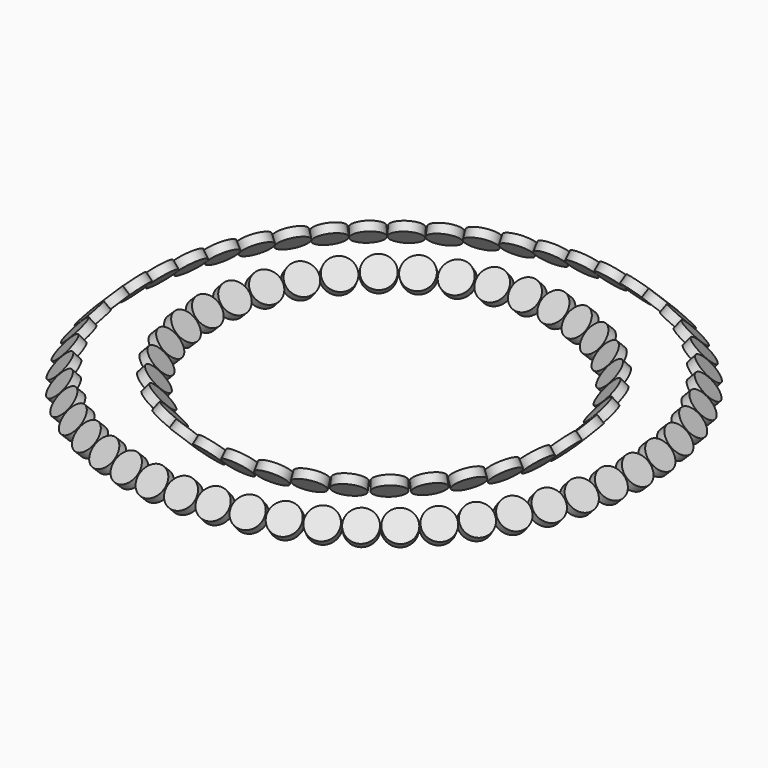
from build123d import *

# Parameters (mm, degrees)
F4_COUNT = 36
F5_COUNT = 52


# Not quite as in the source:
# - the program builds the solid bodies; features that only make, move or delete a surface that nothing else refers to are left out


with BuildPart() as f2:
    # F0 (on Front) → F2 (revolve)
    with BuildSketch(Plane.XZ):
        Polygon((-84.6237436867, 5.7022600949), (-88.1592775926, 2.166726189), (-86.9925514037, 1), (-83.4570174977, 4.5355339059), align=None)
        Polygon((-89.1138717472, 3.1213203436), (-88.1592775926, 2.166726189), (-84.6237436867, 5.7022600949), (-85.5783378413, 6.6568542495), align=None)
    revolve(axis=Axis((-84.0403805922, 0, 5.1188970004), (-0.7071067812, 0, 0.7071067812)))


with BuildPart() as f3:
    # F0 (on Front) → F3 (revolve)
    with BuildSketch(Plane.XZ):
        Polygon((-58.0074485963, 1), (-56.8407224074, 2.166726189), (-60.3762563133, 5.7022600949), (-61.5429825023, 4.5355339059), align=None)
        Polygon((-60.3762563133, 5.7022600949), (-56.8407224074, 2.166726189), (-55.8861282528, 3.1213203436), (-59.4216621587, 6.6568542495), align=None)
    revolve(axis=Axis((-60.9596194078, 0, 5.1188970004), (0.7071067812, 0, 0.7071067812)))


with BuildPart() as f4_1:
    # F4: instance of F3
    add(f3.part.rotate(Axis((0, 0, 16.5421869606), (0, 0, 1)), 1 * 360 / F4_COUNT))


with BuildPart() as f4_2:
    # F4: instance of F3
    add(f3.part.rotate(Axis((0, 0, 16.5421869606), (0, 0, 1)), 2 * 360 / F4_COUNT))


with BuildPart() as f4_3:
    # F4: instance of F3
    add(f3.part.rotate(Axis((0, 0, 16.5421869606), (0, 0, 1)), 3 * 360 / F4_COUNT))


with BuildPart() as f4_4:
    # F4: instance of F3
    add(f3.part.rotate(Axis((0, 0, 16.5421869606), (0, 0, 1)), 4 * 360 / F4_COUNT))


with BuildPart() as f4_5:
    # F4: instance of F3
    add(f3.part.rotate(Axis((0, 0, 16.5421869606), (0, 0, 1)), 5 * 360 / F4_COUNT))


with BuildPart() as f4_6:
    # F4: instance of F3
    add(f3.part.rotate(Axis((0, 0, 16.5421869606), (0, 0, 1)), 6 * 360 / F4_COUNT))


with BuildPart() as f4_7:
    # F4: instance of F3
    add(f3.part.rotate(Axis((0, 0, 16.5421869606), (0, 0, 1)), 7 * 360 / F4_COUNT))


with BuildPart() as f4_8:
    # F4: instance of F3
    add(f3.part.rotate(Axis((0, 0, 16.5421869606), (0, 0, 1)), 8 * 360 / F4_COUNT))


with BuildPart() as f4_9:
    # F4: instance of F3
    add(f3.part.rotate(Axis((0, 0, 16.5421869606), (0, 0, 1)), 9 * 360 / F4_COUNT))


with BuildPart() as f4_10:
    # F4: instance of F3
    add(f3.part.rotate(Axis((0, 0, 16.5421869606), (0, 0, 1)), 10 * 360 / F4_COUNT))


with BuildPart() as f4_11:
    # F4: instance of F3
    add(f3.part.rotate(Axis((0, 0, 16.5421869606), (0, 0, 1)), 11 * 360 / F4_COUNT))


with BuildPart() as f4_12:
    # F4: instance of F3
    add(f3.part.rotate(Axis((0, 0, 16.5421869606), (0, 0, 1)), 12 * 360 / F4_COUNT))


with BuildPart() as f4_13:
    # F4: instance of F3
    add(f3.part.rotate(Axis((0, 0, 16.5421869606), (0, 0, 1)), 13 * 360 / F4_COUNT))


with BuildPart() as f4_14:
    # F4: instance of F3
    add(f3.part.rotate(Axis((0, 0, 16.5421869606), (0, 0, 1)), 14 * 360 / F4_COUNT))


with BuildPart() as f4_15:
    # F4: instance of F3
    add(f3.part.rotate(Axis((0, 0, 16.5421869606), (0, 0, 1)), 15 * 360 / F4_COUNT))


with BuildPart() as f4_16:
    # F4: instance of F3
    add(f3.part.rotate(Axis((0, 0, 16.5421869606), (0, 0, 1)), 16 * 360 / F4_COUNT))


with BuildPart() as f4_17:
    # F4: instance of F3
    add(f3.part.rotate(Axis((0, 0, 16.5421869606), (0, 0, 1)), 17 * 360 / F4_COUNT))


with BuildPart() as f4_18:
    # F4: instance of F3
    add(f3.part.rotate(Axis((0, 0, 16.5421869606), (0, 0, 1)), 18 * 360 / F4_COUNT))


with BuildPart() as f4_19:
    # F4: instance of F3
    add(f3.part.rotate(Axis((0, 0, 16.5421869606), (0, 0, 1)), 19 * 360 / F4_COUNT))


with BuildPart() as f4_20:
    # F4: instance of F3
    add(f3.part.rotate(Axis((0, 0, 16.5421869606), (0, 0, 1)), 20 * 360 / F4_COUNT))


with BuildPart() as f4_21:
    # F4: instance of F3
    add(f3.part.rotate(Axis((0, 0, 16.5421869606), (0, 0, 1)), 21 * 360 / F4_COUNT))


with BuildPart() as f4_22:
    # F4: instance of F3
    add(f3.part.rotate(Axis((0, 0, 16.5421869606), (0, 0, 1)), 22 * 360 / F4_COUNT))


with BuildPart() as f4_23:
    # F4: instance of F3
    add(f3.part.rotate(Axis((0, 0, 16.5421869606), (0, 0, 1)), 23 * 360 / F4_COUNT))


with BuildPart() as f4_24:
    # F4: instance of F3
    add(f3.part.rotate(Axis((0, 0, 16.5421869606), (0, 0, 1)), 24 * 360 / F4_COUNT))


with BuildPart() as f4_25:
    # F4: instance of F3
    add(f3.part.rotate(Axis((0, 0, 16.5421869606), (0, 0, 1)), 25 * 360 / F4_COUNT))


with BuildPart() as f4_26:
    # F4: instance of F3
    add(f3.part.rotate(Axis((0, 0, 16.5421869606), (0, 0, 1)), 26 * 360 / F4_COUNT))


with BuildPart() as f4_27:
    # F4: instance of F3
    add(f3.part.rotate(Axis((0, 0, 16.5421869606), (0, 0, 1)), 27 * 360 / F4_COUNT))


with BuildPart() as f4_28:
    # F4: instance of F3
    add(f3.part.rotate(Axis((0, 0, 16.5421869606), (0, 0, 1)), 28 * 360 / F4_COUNT))


with BuildPart() as f4_29:
    # F4: instance of F3
    add(f3.part.rotate(Axis((0, 0, 16.5421869606), (0, 0, 1)), 29 * 360 / F4_COUNT))


with BuildPart() as f4_30:
    # F4: instance of F3
    add(f3.part.rotate(Axis((0, 0, 16.5421869606), (0, 0, 1)), 30 * 360 / F4_COUNT))


with BuildPart() as f4_31:
    # F4: instance of F3
    add(f3.part.rotate(Axis((0, 0, 16.5421869606), (0, 0, 1)), 31 * 360 / F4_COUNT))


with BuildPart() as f4_32:
    # F4: instance of F3
    add(f3.part.rotate(Axis((0, 0, 16.5421869606), (0, 0, 1)), 32 * 360 / F4_COUNT))


with BuildPart() as f4_33:
    # F4: instance of F3
    add(f3.part.rotate(Axis((0, 0, 16.5421869606), (0, 0, 1)), 33 * 360 / F4_COUNT))


with BuildPart() as f4_34:
    # F4: instance of F3
    add(f3.part.rotate(Axis((0, 0, 16.5421869606), (0, 0, 1)), 34 * 360 / F4_COUNT))


with BuildPart() as f4_35:
    # F4: instance of F3
    add(f3.part.rotate(Axis((0, 0, 16.5421869606), (0, 0, 1)), 35 * 360 / F4_COUNT))


with BuildPart() as f5_1:
    # F5: instance of F2
    add(f2.part.rotate(Axis((0, 0, 16.5421869606), (0, 0, 1)), 1 * 360 / F5_COUNT))


with BuildPart() as f5_2:
    # F5: instance of F2
    add(f2.part.rotate(Axis((0, 0, 16.5421869606), (0, 0, 1)), 2 * 360 / F5_COUNT))


with BuildPart() as f5_3:
    # F5: instance of F2
    add(f2.part.rotate(Axis((0, 0, 16.5421869606), (0, 0, 1)), 3 * 360 / F5_COUNT))


with BuildPart() as f5_4:
    # F5: instance of F2
    add(f2.part.rotate(Axis((0, 0, 16.5421869606), (0, 0, 1)), 4 * 360 / F5_COUNT))


with BuildPart() as f5_5:
    # F5: instance of F2
    add(f2.part.rotate(Axis((0, 0, 16.5421869606), (0, 0, 1)), 5 * 360 / F5_COUNT))


with BuildPart() as f5_6:
    # F5: instance of F2
    add(f2.part.rotate(Axis((0, 0, 16.5421869606), (0, 0, 1)), 6 * 360 / F5_COUNT))


with BuildPart() as f5_7:
    # F5: instance of F2
    add(f2.part.rotate(Axis((0, 0, 16.5421869606), (0, 0, 1)), 7 * 360 / F5_COUNT))


with BuildPart() as f5_8:
    # F5: instance of F2
    add(f2.part.rotate(Axis((0, 0, 16.5421869606), (0, 0, 1)), 8 * 360 / F5_COUNT))


with BuildPart() as f5_9:
    # F5: instance of F2
    add(f2.part.rotate(Axis((0, 0, 16.5421869606), (0, 0, 1)), 9 * 360 / F5_COUNT))


with BuildPart() as f5_10:
    # F5: instance of F2
    add(f2.part.rotate(Axis((0, 0, 16.5421869606), (0, 0, 1)), 10 * 360 / F5_COUNT))


with BuildPart() as f5_11:
    # F5: instance of F2
    add(f2.part.rotate(Axis((0, 0, 16.5421869606), (0, 0, 1)), 11 * 360 / F5_COUNT))


with BuildPart() as f5_12:
    # F5: instance of F2
    add(f2.part.rotate(Axis((0, 0, 16.5421869606), (0, 0, 1)), 12 * 360 / F5_COUNT))


with BuildPart() as f5_13:
    # F5: instance of F2
    add(f2.part.rotate(Axis((0, 0, 16.5421869606), (0, 0, 1)), 13 * 360 / F5_COUNT))


with BuildPart() as f5_14:
    # F5: instance of F2
    add(f2.part.rotate(Axis((0, 0, 16.5421869606), (0, 0, 1)), 14 * 360 / F5_COUNT))


with BuildPart() as f5_15:
    # F5: instance of F2
    add(f2.part.rotate(Axis((0, 0, 16.5421869606), (0, 0, 1)), 15 * 360 / F5_COUNT))


with BuildPart() as f5_16:
    # F5: instance of F2
    add(f2.part.rotate(Axis((0, 0, 16.5421869606), (0, 0, 1)), 16 * 360 / F5_COUNT))


with BuildPart() as f5_17:
    # F5: instance of F2
    add(f2.part.rotate(Axis((0, 0, 16.5421869606), (0, 0, 1)), 17 * 360 / F5_COUNT))


with BuildPart() as f5_18:
    # F5: instance of F2
    add(f2.part.rotate(Axis((0, 0, 16.5421869606), (0, 0, 1)), 18 * 360 / F5_COUNT))


with BuildPart() as f5_19:
    # F5: instance of F2
    add(f2.part.rotate(Axis((0, 0, 16.5421869606), (0, 0, 1)), 19 * 360 / F5_COUNT))


with BuildPart() as f5_20:
    # F5: instance of F2
    add(f2.part.rotate(Axis((0, 0, 16.5421869606), (0, 0, 1)), 20 * 360 / F5_COUNT))


with BuildPart() as f5_21:
    # F5: instance of F2
    add(f2.part.rotate(Axis((0, 0, 16.5421869606), (0, 0, 1)), 21 * 360 / F5_COUNT))


with BuildPart() as f5_22:
    # F5: instance of F2
    add(f2.part.rotate(Axis((0, 0, 16.5421869606), (0, 0, 1)), 22 * 360 / F5_COUNT))


with BuildPart() as f5_23:
    # F5: instance of F2
    add(f2.part.rotate(Axis((0, 0, 16.5421869606), (0, 0, 1)), 23 * 360 / F5_COUNT))


with BuildPart() as f5_24:
    # F5: instance of F2
    add(f2.part.rotate(Axis((0, 0, 16.5421869606), (0, 0, 1)), 24 * 360 / F5_COUNT))


with BuildPart() as f5_25:
    # F5: instance of F2
    add(f2.part.rotate(Axis((0, 0, 16.5421869606), (0, 0, 1)), 25 * 360 / F5_COUNT))


with BuildPart() as f5_26:
    # F5: instance of F2
    add(f2.part.rotate(Axis((0, 0, 16.5421869606), (0, 0, 1)), 26 * 360 / F5_COUNT))


with BuildPart() as f5_27:
    # F5: instance of F2
    add(f2.part.rotate(Axis((0, 0, 16.5421869606), (0, 0, 1)), 27 * 360 / F5_COUNT))


with BuildPart() as f5_28:
    # F5: instance of F2
    add(f2.part.rotate(Axis((0, 0, 16.5421869606), (0, 0, 1)), 28 * 360 / F5_COUNT))


with BuildPart() as f5_29:
    # F5: instance of F2
    add(f2.part.rotate(Axis((0, 0, 16.5421869606), (0, 0, 1)), 29 * 360 / F5_COUNT))


with BuildPart() as f5_30:
    # F5: instance of F2
    add(f2.part.rotate(Axis((0, 0, 16.5421869606), (0, 0, 1)), 30 * 360 / F5_COUNT))


with BuildPart() as f5_31:
    # F5: instance of F2
    add(f2.part.rotate(Axis((0, 0, 16.5421869606), (0, 0, 1)), 31 * 360 / F5_COUNT))


with BuildPart() as f5_32:
    # F5: instance of F2
    add(f2.part.rotate(Axis((0, 0, 16.5421869606), (0, 0, 1)), 32 * 360 / F5_COUNT))


with BuildPart() as f5_33:
    # F5: instance of F2
    add(f2.part.rotate(Axis((0, 0, 16.5421869606), (0, 0, 1)), 33 * 360 / F5_COUNT))


with BuildPart() as f5_34:
    # F5: instance of F2
    add(f2.part.rotate(Axis((0, 0, 16.5421869606), (0, 0, 1)), 34 * 360 / F5_COUNT))


with BuildPart() as f5_35:
    # F5: instance of F2
    add(f2.part.rotate(Axis((0, 0, 16.5421869606), (0, 0, 1)), 35 * 360 / F5_COUNT))


with BuildPart() as f5_36:
    # F5: instance of F2
    add(f2.part.rotate(Axis((0, 0, 16.5421869606), (0, 0, 1)), 36 * 360 / F5_COUNT))


with BuildPart() as f5_37:
    # F5: instance of F2
    add(f2.part.rotate(Axis((0, 0, 16.5421869606), (0, 0, 1)), 37 * 360 / F5_COUNT))


with BuildPart() as f5_38:
    # F5: instance of F2
    add(f2.part.rotate(Axis((0, 0, 16.5421869606), (0, 0, 1)), 38 * 360 / F5_COUNT))


with BuildPart() as f5_39:
    # F5: instance of F2
    add(f2.part.rotate(Axis((0, 0, 16.5421869606), (0, 0, 1)), 39 * 360 / F5_COUNT))


with BuildPart() as f5_40:
    # F5: instance of F2
    add(f2.part.rotate(Axis((0, 0, 16.5421869606), (0, 0, 1)), 40 * 360 / F5_COUNT))


with BuildPart() as f5_41:
    # F5: instance of F2
    add(f2.part.rotate(Axis((0, 0, 16.5421869606), (0, 0, 1)), 41 * 360 / F5_COUNT))


with BuildPart() as f5_42:
    # F5: instance of F2
    add(f2.part.rotate(Axis((0, 0, 16.5421869606), (0, 0, 1)), 42 * 360 / F5_COUNT))


with BuildPart() as f5_43:
    # F5: instance of F2
    add(f2.part.rotate(Axis((0, 0, 16.5421869606), (0, 0, 1)), 43 * 360 / F5_COUNT))


with BuildPart() as f5_44:
    # F5: instance of F2
    add(f2.part.rotate(Axis((0, 0, 16.5421869606), (0, 0, 1)), 44 * 360 / F5_COUNT))


with BuildPart() as f5_45:
    # F5: instance of F2
    add(f2.part.rotate(Axis((0, 0, 16.5421869606), (0, 0, 1)), 45 * 360 / F5_COUNT))


with BuildPart() as f5_46:
    # F5: instance of F2
    add(f2.part.rotate(Axis((0, 0, 16.5421869606), (0, 0, 1)), 46 * 360 / F5_COUNT))


with BuildPart() as f5_47:
    # F5: instance of F2
    add(f2.part.rotate(Axis((0, 0, 16.5421869606), (0, 0, 1)), 47 * 360 / F5_COUNT))


with BuildPart() as f5_48:
    # F5: instance of F2
    add(f2.part.rotate(Axis((0, 0, 16.5421869606), (0, 0, 1)), 48 * 360 / F5_COUNT))


with BuildPart() as f5_49:
    # F5: instance of F2
    add(f2.part.rotate(Axis((0, 0, 16.5421869606), (0, 0, 1)), 49 * 360 / F5_COUNT))


with BuildPart() as f5_50:
    # F5: instance of F2
    add(f2.part.rotate(Axis((0, 0, 16.5421869606), (0, 0, 1)), 50 * 360 / F5_COUNT))


with BuildPart() as f5_51:
    # F5: instance of F2
    add(f2.part.rotate(Axis((0, 0, 16.5421869606), (0, 0, 1)), 51 * 360 / F5_COUNT))


solid = Compound([f2.part, f3.part, f4_1.part, f4_2.part, f4_3.part, f4_4.part, f4_5.part, f4_6.part, f4_7.part, f4_8.part, f4_9.part, f4_10.part, f4_11.part, f4_12.part, f4_13.part, f4_14.part, f4_15.part, f4_16.part, f4_17.part, f4_18.part, f4_19.part, f4_20.part, f4_21.part, f4_22.part, f4_23.part, f4_24.part, f4_25.part, f4_26.part, f4_27.part, f4_28.part, f4_29.part, f4_30.part, f4_31.part, f4_32.part, f4_33.part, f4_34.part, f4_35.part, f5_1.part, f5_2.part, f5_3.part, f5_4.part, f5_5.part, f5_6.part, f5_7.part, f5_8.part, f5_9.part, f5_10.part, f5_11.part, f5_12.part, f5_13.part, f5_14.part, f5_15.part, f5_16.part, f5_17.part, f5_18.part, f5_19.part, f5_20.part, f5_21.part, f5_22.part, f5_23.part, f5_24.part, f5_25.part, f5_26.part, f5_27.part, f5_28.part, f5_29.part, f5_30.part, f5_31.part, f5_32.part, f5_33.part, f5_34.part, f5_35.part, f5_36.part, f5_37.part, f5_38.part, f5_39.part, f5_40.part, f5_41.part, f5_42.part, f5_43.part, f5_44.part, f5_45.part, f5_46.part, f5_47.part, f5_48.part, f5_49.part, f5_50.part, f5_51.part])
